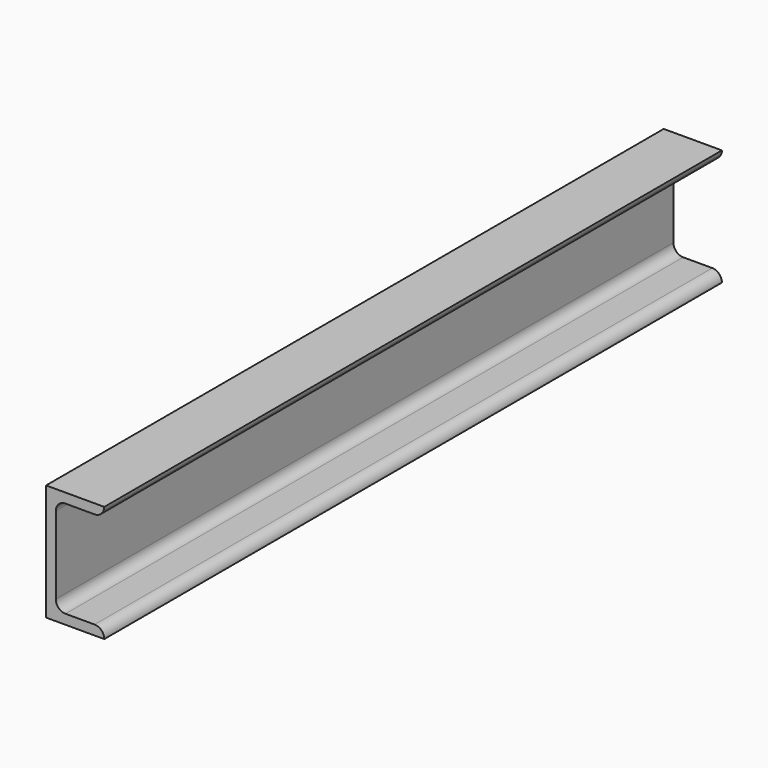
from build123d import *

# Parameters (mm, degrees)
F1_DEPTH = 505.46


# Not quite as in the source:
# - ends of sketch curves that miss each other by under 0.0002 mm in the source are joined


with BuildPart() as f1:
    # F0 (on Front) → F1 (new body)
    with BuildSketch(Plane.XZ):
        with BuildLine():
            Line((0, 76.2), (0, 0))
            Line((0, 0), (38.1, 0))
            ThreePointArc((38.1, 0), (36.2401280605, 4.4901312434), (31.75, 6.3500031829))
            Line((31.75, 6.3500031829), (12.7000031829, 6.3500031829))
            ThreePointArc((12.7000031829, 6.3500031829), (8.2098751224, 8.2098751224), (6.3500031829, 12.7000031829))
            Line((6.3500031829, 12.7000031829), (6.3500031829, 63.4999968171))
            ThreePointArc((6.3500031829, 63.4999968171), (8.2098751224, 67.9901248776), (12.7000031829, 69.8499968171))
            Line((12.7000031829, 69.8499968171), (31.75, 69.8499968171))
            ThreePointArc((31.75, 69.8499968171), (36.2401280605, 71.7098687566), (38.1, 76.1999968171))
            Line((38.1, 76.1999968171), (0, 76.2))
        make_face()
    extrude(amount=F1_DEPTH)


solid = f1.part
